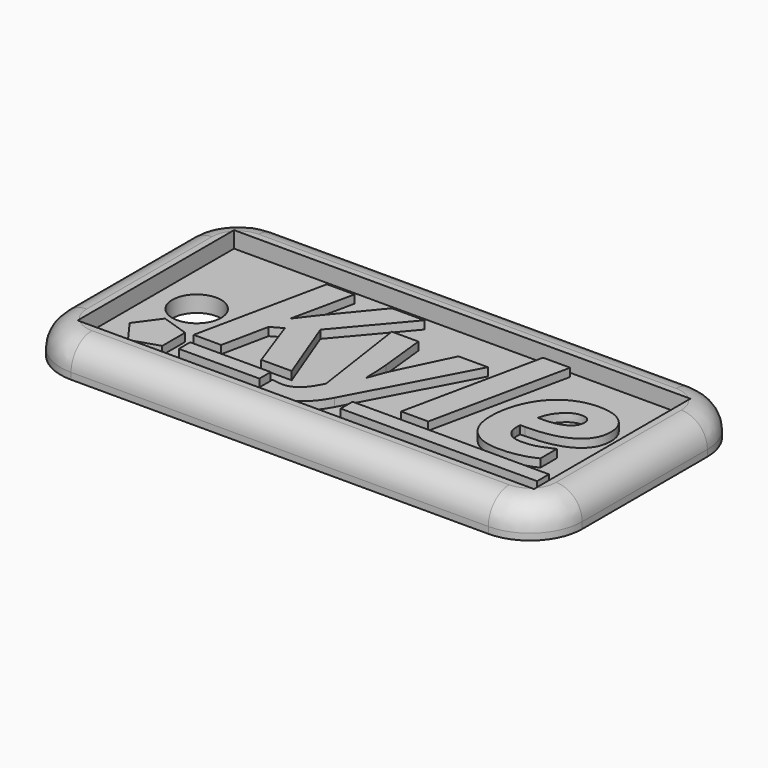
from build123d import *

# Parameters (mm, degrees)
F0_W         = 44.45
F0_H         = 19.05
F0_R         = 2.38125
F1_DEPTH     = 1.5875
F0_W_2       = 50.8
F0_H_2       = 25.4
F2_DEPTH     = 3.175
F3_R         = 5.08
F4_T1_DEPTH  = 40.64
F4_T3_DEPTH  = 15.24
F4_T6_ANGLE  = 90
F4_T8_ANGLE  = 90
F4_T10_ANGLE = 90
F4_T12_ANGLE = 90
F5_W         = 7.8462520614
F5_H         = 1.3765357435
F5_W_2       = 19.1338453442
F5_H_2       = 1.4453623444
F5_TEXT_SIZE = 17.975046972
F6_DEPTH     = 0.79375
F7_DEPTH     = 0.79375
F8_DEPTH     = 0.79375


# Not quite as in the source:
# - a fillet or chamfer that OpenCascade refuses, or shapes differently, is made with other operations: its cross-section is extruded or revolved along the edge and cut away or added
# - Text() gives the source's letters only with a copy of the font that has no kerning and outlines rounded to 1/6400 em; it was checked with that copy


with BuildPart() as f1:
    # F0 (on Top) → F1 (new body)
    with BuildSketch(Plane.XY):
        with Locations((25.4, 12.7)):
            Rectangle(F0_W, F0_H)
        with Locations((7.15645, 12.7)):
            Circle(F0_R, mode=Mode.SUBTRACT)
    extrude(amount=F1_DEPTH)

    # F0 (on Top) → F2 (join)
    with BuildSketch(Plane.XY):
        with Locations((25.4, 12.7)):
            Rectangle(F0_W_2, F0_H_2)
        with Locations((25.4, 12.7)):
            Rectangle(F0_W, F0_H, mode=Mode.SUBTRACT)
    extrude(amount=F2_DEPTH)

    # F3
    f3_edges = [f1.edges().sort_by_distance(p)[0] for p in [
        (50.8, 0, 1.5875),
        (50.8, 25.4, 1.5875),
        (0, 25.4, 1.5875),
        (0, 0, 1.5875),
    ]]
    fillet(f3_edges, radius=F3_R)

    # F4: fillet of radius 2.54 on 8 edges, made by hand

    # F4_s2 → F4_t1 (cut)
    with BuildSketch(Plane.YZ.offset(5.08)):
        with BuildLine():
            ThreePointArc((25.4, 0.635), (24.6560512242, 2.4310512242), (22.86, 3.175))
            Line((22.86, 3.175), (25.4, 3.175))
            Line((25.4, 3.175), (25.4, 0.635))
        make_face()
        with BuildLine():
            ThreePointArc((0, 0.635), (0.7439487758, 2.4310512242), (2.54, 3.175))
            Line((2.54, 3.175), (0, 3.175))
            Line((0, 3.175), (0, 0.635))
        make_face()
    extrude(amount=F4_T1_DEPTH, mode=Mode.SUBTRACT)

    # F4_s4 → F4_t3 (cut)
    with BuildSketch(Plane.XZ.offset(-20.32)):
        with BuildLine():
            ThreePointArc((0, 0.635), (0.7439487758, 2.4310512242), (2.54, 3.175))
            Line((2.54, 3.175), (0, 3.175))
            Line((0, 3.175), (0, 0.635))
        make_face()
        with BuildLine():
            ThreePointArc((50.8, 0.635), (50.0560512242, 2.4310512242), (48.26, 3.175))
            Line((48.26, 3.175), (50.8, 3.175))
            Line((50.8, 3.175), (50.8, 0.635))
        make_face()
    extrude(amount=F4_T3_DEPTH, mode=Mode.SUBTRACT)

    # F4_s5 → F4_t6 (revolve, cut)
    with BuildSketch(Plane.XZ.offset(-20.32)):
        with BuildLine():
            ThreePointArc((0, 0.635), (0.7439487758, 2.4310512242), (2.54, 3.175))
            Line((2.54, 3.175), (0, 3.175))
            Line((0, 3.175), (0, 0.635))
        make_face()
    revolve(axis=Axis((5.08, 20.32, 3.175), (0, 0, -1)), revolution_arc=F4_T6_ANGLE, mode=Mode.SUBTRACT)

    # F4_s7 → F4_t8 (revolve, cut)
    with BuildSketch(Plane.XZ.offset(-5.08)):
        with BuildLine():
            ThreePointArc((0, 0.635), (0.7439487758, 2.4310512242), (2.54, 3.175))
            Line((2.54, 3.175), (0, 3.175))
            Line((0, 3.175), (0, 0.635))
        make_face()
    revolve(axis=Axis((5.08, 5.08, 3.175), (0, 0, 1)), revolution_arc=F4_T8_ANGLE, mode=Mode.SUBTRACT)

    # F4_s9 → F4_t10 (revolve, cut)
    with BuildSketch(Plane.XZ.offset(-20.32)):
        with BuildLine():
            ThreePointArc((50.8, 0.635), (50.0560512242, 2.4310512242), (48.26, 3.175))
            Line((48.26, 3.175), (50.8, 3.175))
            Line((50.8, 3.175), (50.8, 0.635))
        make_face()
    revolve(axis=Axis((45.72, 20.32, 3.175), (0, 0, 1)), revolution_arc=F4_T10_ANGLE, mode=Mode.SUBTRACT)

    # F4_s11 → F4_t12 (revolve, cut)
    with BuildSketch(Plane.YZ.offset(45.72)):
        with BuildLine():
            ThreePointArc((0, 0.635), (0.7439487758, 2.4310512242), (2.54, 3.175))
            Line((2.54, 3.175), (0, 3.175))
            Line((0, 3.175), (0, 0.635))
        make_face()
    revolve(axis=Axis((45.72, 5.08, 3.175), (0, 0, 1)), revolution_arc=F4_T12_ANGLE, mode=Mode.SUBTRACT)

    # F5 (on face) → F6 (join)
    with BuildSketch(Plane.XY.offset(1.5875)):
        Polygon((9.8692663014, 5.1128118639), (9.8692663014, 7.898819692), (7.219615402, 8.7597434573), (5.5820410879, 6.5058157779), (7.219615402, 4.2518880985), align=None)
        with Locations((15.0806005113, 6.2131495215)):
            Rectangle(F5_W, F5_H)
        with Locations((36.4857306704, 6.247562822)):
            Rectangle(F5_W_2, F5_H_2)
        with Locations((10.1331500337, 8.0302460119)):
            Text('Kyle', F5_TEXT_SIZE, font='Open Sans', font_style=FontStyle.BOLDITALIC, text_align=(TextAlign.LEFT, TextAlign.BOTTOM))
    extrude(amount=F6_DEPTH)

    # F5 (on face) → F7 (join)
    with BuildSketch(Plane.XY.offset(1.5875)):
        Polygon((9.8692663014, 5.1128118639), (9.8692663014, 7.898819692), (7.219615402, 8.7597434573), (5.5820410879, 6.5058157779), (7.219615402, 4.2518880985), align=None)
        with Locations((15.0806005113, 6.2131495215)):
            Rectangle(F5_W, F5_H)
        with Locations((36.4857306704, 6.247562822)):
            Rectangle(F5_W_2, F5_H_2)
        with Locations((10.1331500337, 8.0302460119)):
            Text('Kyle', F5_TEXT_SIZE, font='Open Sans', font_style=FontStyle.BOLDITALIC, text_align=(TextAlign.LEFT, TextAlign.BOTTOM))
    extrude(amount=F7_DEPTH)

    # F5 (on face) → F8 (join)
    with BuildSketch(Plane.XY.offset(1.5875)):
        Polygon((9.8692663014, 5.1128118639), (9.8692663014, 7.898819692), (7.219615402, 8.7597434573), (5.5820410879, 6.5058157779), (7.219615402, 4.2518880985), align=None)
        with Locations((15.0806005113, 6.2131495215)):
            Rectangle(F5_W, F5_H)
        with Locations((36.4857306704, 6.247562822)):
            Rectangle(F5_W_2, F5_H_2)
        with Locations((10.1331500337, 8.0302460119)):
            Text('Kyle', F5_TEXT_SIZE, font='Open Sans', font_style=FontStyle.BOLDITALIC, text_align=(TextAlign.LEFT, TextAlign.BOTTOM))
    extrude(amount=F8_DEPTH)


solid = f1.part
